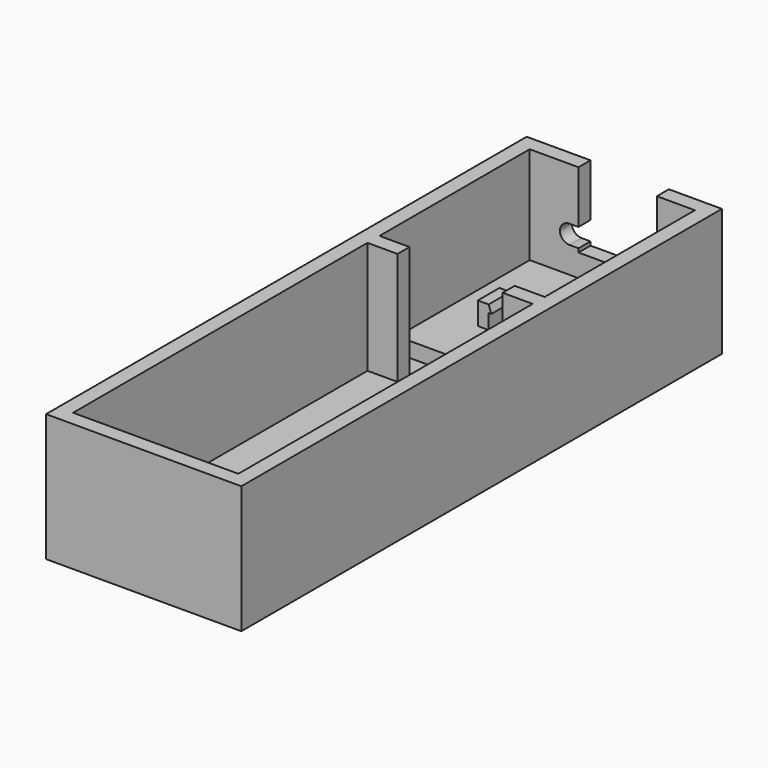
from build123d import *

# Parameters (mm, degrees)
F0_W        = 33.02
F0_H        = 101.6
F1_DEPTH    = 2.54
F2_W        = 33.02
F2_H        = 101.6
F2_W_2      = 5.08
F2_H_2      = 2.54
F3_DEPTH    = 19.05
F2_W_3      = 27.94
F2_H_3      = 27.94
F2_W_4      = 1.8288
F2_H_4      = 4.572
F4_DEPTH    = 2.54
F5_DEPTH    = 5.08
F7_W        = 3.1588217151
F7_H        = 3.175
F8_DEPTH    = 25.4
F9_T1_DEPTH = 2.54
F10_W       = 0.4572
F10_H       = 4.572
F10_W_2     = 1.8288
F10_W_3     = 2.286
F11_DEPTH   = 1.27
F13_DEPTH   = 6.35


# Not quite as in the source:
# - a fillet or chamfer that OpenCascade refuses, or shapes differently, is made with other operations: its cross-section is extruded or revolved along the edge and cut away or added


with BuildPart() as f1:
    # F0 (on Top) → F1 (new body)
    with BuildSketch(Plane.XY):
        with Locations((16.51, 50.8)):
            Rectangle(F0_W, F0_H)
    extrude(amount=F1_DEPTH)

    # F2 (on face) → F3 (join)
    with BuildSketch(Plane.XY.offset(2.54)):
        with Locations((16.51, 50.8)):
            Rectangle(F2_W, F2_H)
        Polygon((30.48, 2.54), (2.54, 2.54), (2.54, 64.77), (2.54, 67.31), (2.54, 71.12), (2.54, 99.06), (30.48, 99.06), (30.48, 71.12), (30.48, 67.31), (30.48, 64.77), align=None, mode=Mode.SUBTRACT)
        with Locations((5.08, 66.04)):
            Rectangle(F2_W_2, F2_H_2)
        with Locations((27.94, 66.04)):
            Rectangle(F2_W_2, F2_H_2)
    extrude(amount=F3_DEPTH)

    # F2 (on face) → F4 (join)
    with BuildSketch(Plane.XY.offset(2.54)):
        with Locations((16.51, 85.09)):
            Rectangle(F2_W_3, F2_H_3)
        with Locations((9.8806, 82.3468)):
            Rectangle(F2_W_4, F2_H_4, mode=Mode.SUBTRACT)
        with Locations((23.1394, 82.3468)):
            Rectangle(F2_W_4, F2_H_4, mode=Mode.SUBTRACT)
    extrude(amount=F4_DEPTH)

    # F2 (on face) → F5 (join)
    with BuildSketch(Plane.XY.offset(2.54)):
        with Locations((9.8806, 82.3468)):
            Rectangle(F2_W_4, F2_H_4)
        with Locations((23.1394, 82.3468)):
            Rectangle(F2_W_4, F2_H_4)
    extrude(amount=F5_DEPTH)

    # F7 (on face) → F8 (cut)
    with BuildSketch(Plane.XZ.offset(-99.06)):
        Polygon((10.795, 9.525), (10.795, 8.89), (24.0538, 8.89), (24.0538, 21.59), (10.795, 21.59), (10.795, 12.7), align=None)
        with Locations((9.2155891424, 11.1125)):
            Rectangle(F7_W, F7_H)
    extrude(amount=-F8_DEPTH, mode=Mode.SUBTRACT)

    # F9: fillet of radius 1.651 on 2 edges, made by hand

    # F9_s2 → F9_t1 (join)
    with BuildSketch(Plane.XZ.offset(-101.6)):
        with BuildLine():
            ThreePointArc((9.2871782849, 12.7), (8.1197449891, 12.2164332957), (7.6361782849, 11.049))
            Line((7.6361782849, 11.049), (7.6361782849, 12.7))
            Line((7.6361782849, 12.7), (9.2871782849, 12.7))
        make_face()
        with BuildLine():
            ThreePointArc((7.6361782849, 11.176), (8.1197449891, 10.0085667043), (9.2871782849, 9.525))
            Line((9.2871782849, 9.525), (7.6361782849, 9.525))
            Line((7.6361782849, 9.525), (7.6361782849, 11.176))
        make_face()
    extrude(amount=F9_T1_DEPTH)

    # F10 (on face) → F11 (join)
    with BuildSketch(Plane.XY.offset(7.62)):
        with Locations((11.0236, 82.3468)):
            Rectangle(F10_W, F10_H)
        with Locations((9.8806, 82.3468)):
            Rectangle(F10_W_2, F10_H)
        with Locations((22.9108, 82.3468)):
            Rectangle(F10_W_3, F10_H)
    extrude(amount=F11_DEPTH)

    # F12 (on face) → F13 (cut)
    with BuildSketch(Plane.XZ.offset(-80.0608)):
        Polygon((10.795, 8.89), (11.2522, 7.62), (11.2522, 8.89), align=None)
        Polygon((21.7678, 7.62), (22.225, 8.89), (21.7678, 8.89), align=None)
    extrude(amount=-F13_DEPTH, mode=Mode.SUBTRACT)


solid = f1.part
